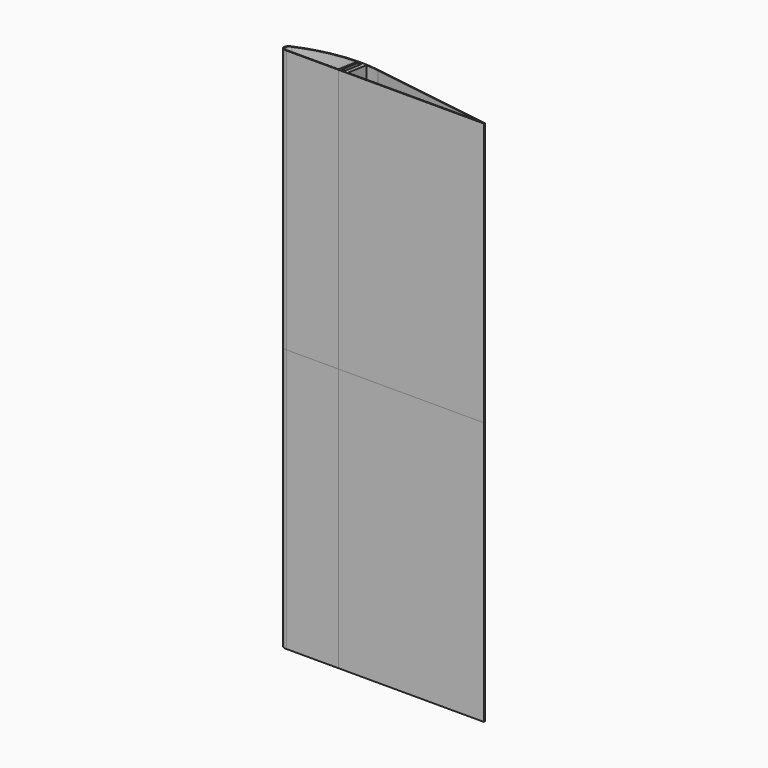
from build123d import *

# Parameters (mm, degrees)
F1_DEPTH     = 200
F3_DEPTH     = 200
F4_T         = -0.8
F4_2_T       = -0.8
F5_W         = 2.5
F5_H         = 1
F6_DEPTH     = 20
F7_T4_DEPTH  = 5.5
F7_T9_DEPTH  = 30.5
F7_T14_ANGLE = 37.7423343373
F7_T20_ANGLE = 37.7423343373
F8_W         = 155.1876314091
F8_H         = 22.3366669118
F9_ANGLE     = 7


# Not quite as in the source:
# - a fillet or chamfer that OpenCascade refuses, or shapes differently, is made with other operations: its cross-section is extruded or revolved along the edge and cut away or added


with BuildPart() as f1:
    # F0 (on Top) → F1 (new body)
    with BuildSketch(Plane.XY):
        with BuildLine():
            Line((94.1401966023, -3), (94.1696608117, -2.0004341641))
            Line((94.1696608117, -2.0004341641), (0, 15))
            ThreePointArc((0, 15), (-7.9879059152, 16.0504323354), (-16.0396361483, 16.3327251865))
            Line((-16.0396361483, 16.3327251865), (-16.0396361483, -3))
            Line((-16.0396361483, -3), (94.1401966023, -3))
        make_face()
    extrude(amount=F1_DEPTH)

    # F4
    f4_openings = [f1.faces().sort_by_distance(p)[0] for p in [
        (22.614044, 3.891358, 200),
    ]]
    offset(amount=F4_T, openings=f4_openings)

    # F5 (on face) → F6 (join)
    with BuildSketch(Plane.XY.offset(200)):
        Polygon((-12.7396361483, -1.2), (-12.7396361483, -2.2), (-9.7396361483, -2.2), (-9.7396361483, 15.5391672506), (-12.7396361483, 15.5391672506), (-12.7396361483, 14.5391672506), align=None)
        with Locations((-13.9896361483, -1.7)):
            Rectangle(F5_W, F5_H)
        with Locations((-13.9896361483, 15.0391672506)):
            Rectangle(F5_W, F5_H)
    extrude(amount=-F6_DEPTH)

    # F7: fillet of radius 10 on 2 edges, made by hand


with BuildPart() as f3:
    # F2 (on face) → F3 (new body)
    with BuildSketch(Plane.XY.offset(200)):
        with BuildLine():
            Line((-16.0396361483, -3), (-16.0396361483, 16.3327251865))
            ThreePointArc((-16.0396361483, 16.3327251865), (-37.5222437907, 13.2612199418), (-57.5066562048, 4.8019152395))
            ThreePointArc((-57.5066562048, 4.8019152395), (-60.2806962129, 0.1415930949), (-55.8598033977, -3))
            Line((-55.8598033977, -3), (-16.0396361483, -3))
        make_face()
    extrude(amount=-F3_DEPTH)

    # F4#2
    f4_2_openings = [f3.faces().sort_by_distance(p)[0] for p in [
        (-34.83961, 5.023506, 200),
    ]]
    offset(amount=F4_2_T, openings=f4_2_openings, kind=Kind.INTERSECTION)


with BuildPart() as f7_tool2:
    # F7_s3 → F7_t4 (new body)
    with BuildSketch(Plane.YZ.offset(-15.2396361483)):
        with BuildLine():
            ThreePointArc((-2.2, 170), (0.7289321881, 177.0710678119), (7.8, 180))
            Line((7.8, 180), (-2.2, 180))
            Line((-2.2, 180), (-2.2, 170))
        make_face()
    extrude(amount=F7_T4_DEPTH)

    split(bisect_by=Plane.XZ.offset(1.2), keep=Keep.TOP)


with BuildPart() as f1_1:
    add(f1.part)

    # F7_t1: union F7_tool2
    add(f7_tool2.part)


with BuildPart() as f7_tool7:
    # F7_s8 → F7_t9 (new body)
    with BuildSketch(Plane.YZ.offset(-40.2396361483)):
        with BuildLine():
            ThreePointArc((-2.2, 170), (0.7289321881, 177.0710678119), (7.8, 180))
            Line((7.8, 180), (-2.2, 180))
            Line((-2.2, 180), (-2.2, 170))
        make_face()
    extrude(amount=F7_T9_DEPTH)

    split(bisect_by=Plane.YZ.offset(-12.7396361483), keep=Keep.TOP)


with BuildPart() as f1_2:
    add(f1_1.part)

    # F7_t6: union F7_tool7
    add(f7_tool7.part)


with BuildPart() as f7_tool12:
    # F7_s13 → F7_t14 (revolve)
    with BuildSketch(Plane(origin=(-32.6433997569, -9.9682739464, 0), x_dir=(0, 0, 1), z_dir=(-0.9564014883, -0.2920551201, 0))):
        with BuildLine():
            ThreePointArc((170, 22.8682565899), (177.0710678119, 19.9393244018), (180, 12.8682565899))
            Line((180, 12.8682565899), (180, 22.8682565899))
            Line((180, 22.8682565899), (170, 22.8682565899))
        make_face()
    revolve(axis=Axis((-14.9610707823, -67.8731164952, 180), (0, 0, -1)), revolution_arc=F7_T14_ANGLE)

    split(bisect_by=Plane.YZ.offset(-12.7396361483), keep=Keep.TOP)

    split(bisect_by=Plane.YZ.offset(-9.7396361483), keep=Keep.BOTTOM)


with BuildPart() as f1_3:
    add(f1_2.part)

    # F7_t11: union F7_tool12
    add(f7_tool12.part)


with BuildPart() as f7_tool18:
    # F7_s19 → F7_t20 (revolve)
    with BuildSketch(Plane(origin=(-32.6433997569, -9.9682739464, 0), x_dir=(0, 0, 1), z_dir=(-0.9564014883, -0.2920551201, 0))):
        with BuildLine():
            ThreePointArc((170, 22.8682565899), (177.0710678119, 19.9393244018), (180, 12.8682565899))
            Line((180, 12.8682565899), (180, 22.8682565899))
            Line((180, 22.8682565899), (170, 22.8682565899))
        make_face()
    revolve(axis=Axis((-14.9610707823, -67.8731164952, 180), (0, 0, -1)), revolution_arc=F7_T20_ANGLE)

    split(bisect_by=Plane.YZ.offset(-15.2396361483), keep=Keep.TOP)

    split(bisect_by=Plane.XZ.offset(-14.5391672506), keep=Keep.BOTTOM)

    split(bisect_by=Plane.XZ.offset(-15.5391672506), keep=Keep.TOP)

    split(bisect_by=Plane.YZ.offset(-9.7396361483), keep=Keep.BOTTOM)


with BuildPart() as f1_4:
    add(f1_3.part)

    # F7_t17: union F7_tool18
    add(f7_tool18.part)


with BuildPart() as f9_tool:
    # F8 (on face) → F9 (revolve)
    with BuildSketch(Plane.XY.offset(200)):
        with Locations((16.5463808977, 8.1683334559)):
            Rectangle(F8_W, F8_H)
    revolve(axis=Axis((16.5463808977, -3, 200), (-1, 0, 0)), revolution_arc=F9_ANGLE)


with BuildPart() as f1_5:
    add(f1_4.part)

    # F9: cut by f9_tool
    add(f9_tool.part, mode=Mode.SUBTRACT)


with BuildPart() as f3_1:
    add(f3.part)

    # F9: cut by f9_tool
    add(f9_tool.part, mode=Mode.SUBTRACT)


with BuildPart() as f10_1:
    # F10: instance of F1
    add(f1_5.part.mirror(Plane.XY))


with BuildPart() as f10_2:
    # F10: instance of F3
    add(f3_1.part.mirror(Plane.XY))


solid = Compound([f1_5.part, f3_1.part, f10_1.part, f10_2.part])
